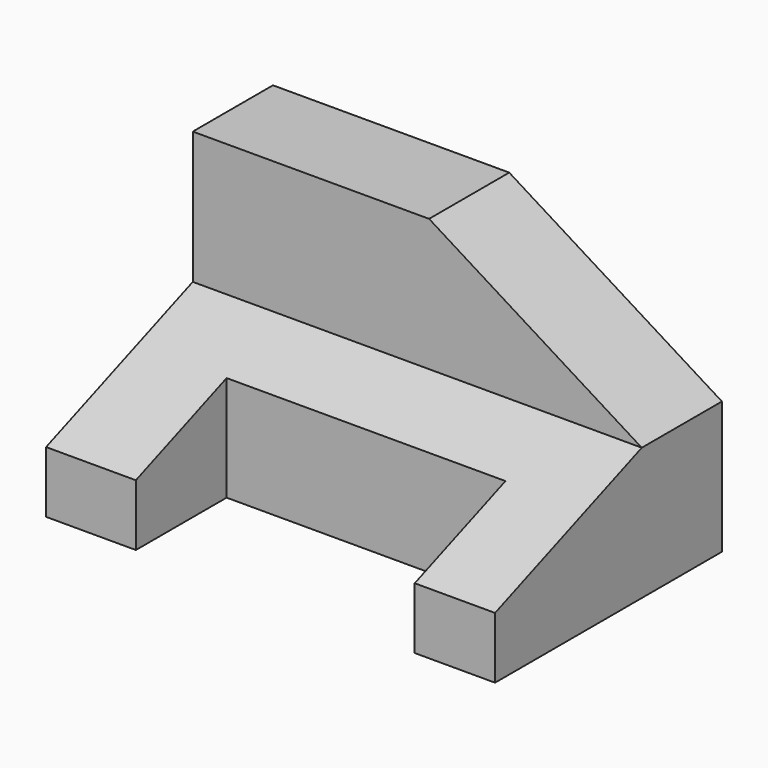
from build123d import *

# Parameters (mm, degrees)
F1_DEPTH = 95
F3_DEPTH = 21.2002830101
F5_DEPTH = 25
F6_W     = 59
F6_H     = 24
F7_DEPTH = 30


with BuildPart() as f1:
    # F0 (on Right) → F1 (new body)
    with BuildSketch(Plane.YZ):
        Polygon((-60, 0), (0, 0), (0, 56), (-21.2002830101, 56), (-21.2002830101, 28), (-60, 13), align=None)
    extrude(amount=-F1_DEPTH)

    # F2 (on face) → F3 (join, through all)
    with BuildSketch(Plane.XZ.offset(21.2002830101)):
        Polygon((0, 56), (-38.8899631798, 56), (0, 28), align=None)
    extrude(amount=-F3_DEPTH)

    # F4 (on face) → F5 (cut)
    with BuildSketch(Plane.XZ.offset(21.2002830101)):
        Polygon((0, 56), (-45, 56), (0, 28), align=None)
    extrude(amount=-F5_DEPTH, mode=Mode.SUBTRACT)

    # F6 (on face) → F7 (cut)
    with BuildSketch(Plane(origin=(0, 0, 0), x_dir=(1, 0, 0), z_dir=(0, 0, -1))):
        with Locations((-46.5, 48)):
            Rectangle(F6_W, F6_H)
    extrude(amount=-F7_DEPTH, mode=Mode.SUBTRACT)


with BuildPart() as f1_1:
    # F8: moved
    add(f1.part.moved(Location((95, 0, 0))))


solid = f1_1.part
